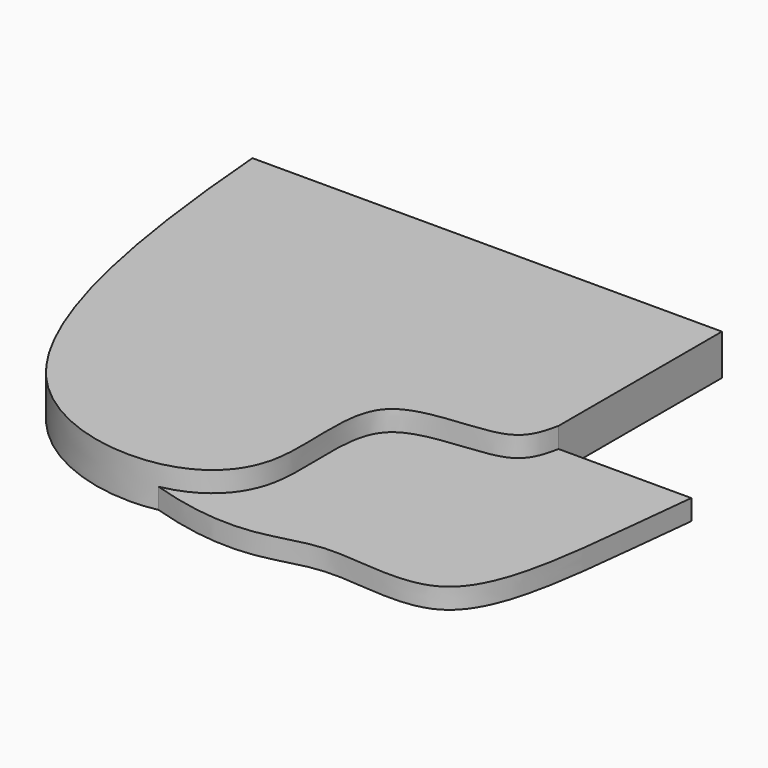
from build123d import *

# Parameters (mm, degrees)
F2_DEPTH = 50.8
F3_DEPTH = 25.4


# Not quite as in the source:
# - the dataset's text gives a spline's control points without its knots; the knots are read off the source's solid


with BuildPart() as f2:
    # F0 (on Top) → F2 (new body)
    with BuildSketch(Plane.XY):
        with BuildLine():
            Line((584.2, 0), (0, 0))
            add(Edge.make_bspline(
                [(0, 0), (15.1486947055, -189.218948528), (65.9452547031, -521.1208855176), (331.2736157203, -584.8076926646), (439.4210233355, -494.812023687), (384.6079093416, -293.977624041), (569.828929238, -318.1440119701), (580.1429311177, -272.0586668), (584.2, -254)],
                knots=[0, 0, 0, 0, 0.2870068182, 0.4704907214, 0.6055466033, 0.7629356749, 0.9076890707, 1, 1, 1, 1], degree=3))
            Line((584.2, -254), (584.2, 0))
        make_face()
    extrude(amount=F2_DEPTH)

    # F1 (on Top) → F3 (join)
    with BuildSketch(Plane.XY):
        with BuildLine():
            add(Edge.make_bspline(
                [(330.2, -558.8), (372.9674701378, -550.1118418504), (439.4210233355, -494.812023687), (384.6079093416, -293.977624041), (569.828929238, -318.1440119701), (580.1429311177, -272.0586668), (584.2, -254)],
                knots=[0.4704907214, 0.4704907214, 0.4704907214, 0.4704907214, 0.6055466033, 0.7629356749, 0.9076890707, 1, 1, 1, 1], degree=3))
            add(Edge.make_bspline(
                [(330.2, -558.8), (389.6603919437, -577.5870896762), (465.8574745229, -582.035806053), (541.2894567383, -546.8586607902), (727.1294826657, -594.3131958041), (732.2998279498, -401.9058890127), (749.3, -254)],
                knots=[0, 0, 0, 0, 0.2368976142, 0.4165860366, 0.6473220038, 1, 1, 1, 1], degree=3))
            Line((749.3, -254), (584.2, -254))
        make_face()
    extrude(amount=F3_DEPTH)


solid = f2.part
